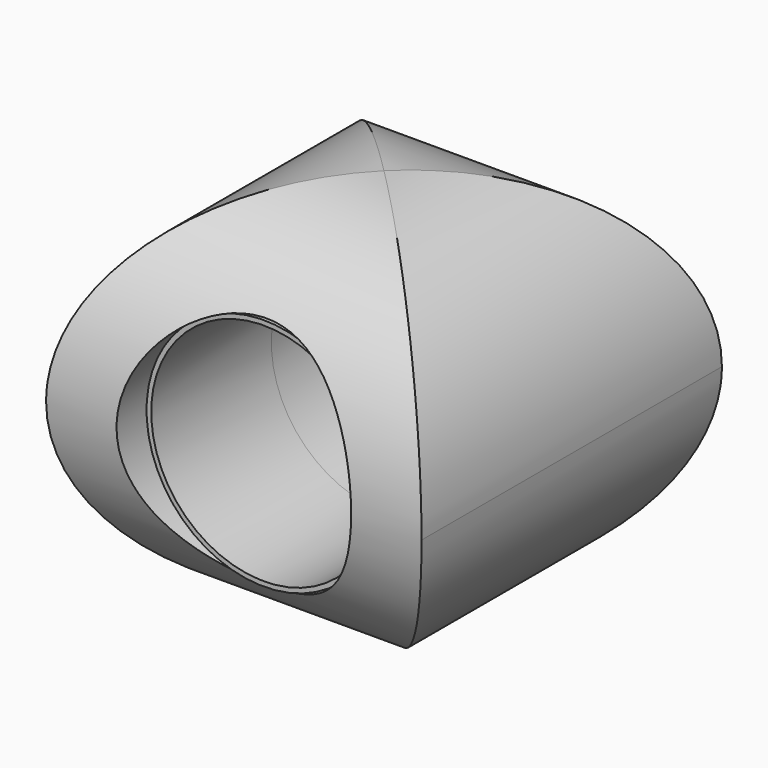
from build123d import *

# Parameters (mm, degrees)
F0_R          = 39.6875
F0_R_2        = 38.1
F2_DEPTH      = 50.8
F2_DEPTH_BACK = 50.8
F1_R          = 63.5
F1_R_2        = 26.9875
F1_R_3        = 25.4
F3_DEPTH      = 63.5
F3_DEPTH_BACK = 63.5
F0_R_3        = 63.5
F6_DEPTH      = 63.5


# Not quite as in the source:
# - a feature of the source that left no trace in its solid (it failed there, or was rolled back) is left out


with BuildPart() as f2:
    # F0 (on Front) → F2 (new body, two sides)
    with BuildSketch(Plane.XZ) as f2_sk:
        Circle(F0_R)
        Circle(F0_R_2, mode=Mode.SUBTRACT)
    extrude(amount=-F2_DEPTH)
    extrude(f2_sk.sketch, amount=F2_DEPTH_BACK)


with BuildPart() as f3:
    # F1 (on Right) → F3 (new body, two sides)
    with BuildSketch(Plane.YZ) as f3_sk:
        Circle(F1_R)
        Circle(F1_R_2, mode=Mode.SUBTRACT)
        Circle(F1_R_2)
        Circle(F1_R_3, mode=Mode.SUBTRACT)
        Circle(F1_R_3)
    extrude(amount=F3_DEPTH)
    extrude(f3_sk.sketch, amount=-F3_DEPTH_BACK)

    # F0 (on Front) → F6 (intersect, symmetric)
    with BuildSketch(Plane.XZ):
        Circle(F0_R_3)
        Circle(F0_R, mode=Mode.SUBTRACT)
    extrude(amount=F6_DEPTH, both=True, mode=Mode.INTERSECT)


solid = Compound([f2.part, f3.part])
